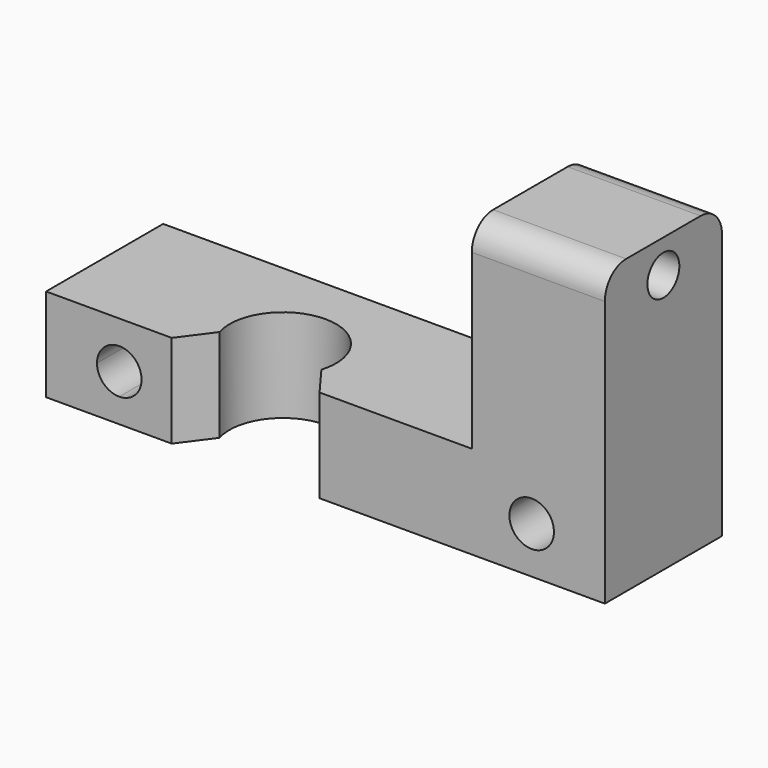
from build123d import *

# Parameters (mm, degrees)
F1_W        = 42
F1_H        = 11
F2_DEPTH    = 7
F3_R        = 4
F4_DEPTH    = 25
F5_T1_DEPTH = 25.9605224852
F7_DEPTH    = 25
F8_W        = 10
F8_H        = 11
F9_DEPTH    = 15
F10_R       = 1.5
F11_DEPTH   = 25
F12_R       = 2


# Not quite as in the source:
# - a fillet or chamfer that OpenCascade refuses, or shapes differently, is made with other operations: its cross-section is extruded or revolved along the edge and cut away or added


with BuildPart() as f2:
    # F1 (on Top) → F2 (new body)
    with BuildSketch(Plane.XY):
        with Locations((21, 5.5)):
            Rectangle(F1_W, F1_H)
    extrude(amount=F2_DEPTH)

    # F3 (on face) → F4 (cut)
    with BuildSketch(Plane.XY.offset(7)):
        with Locations((15, 3.5)):
            Circle(F3_R)
    extrude(amount=-F4_DEPTH, mode=Mode.SUBTRACT)

    # F5: chamfer of 7 on 2 edges, made by hand

    # F5_s2 → F5_t1 (cut)
    with BuildSketch(Plane.XY.offset(-9.4802612426)):
        with BuildLine():
            Line((20.721915214, -0.225000294), (18.6596772309, 2.5591704653))
            Line((18.6596772309, 2.5591704653), (18.5257555, 2.5999745093))
            ThreePointArc((18.5257555, 2.5999745093), (18.0236462707, 1.1005910665), (16.8687144645, 0.1225))
            Line((16.8687144645, 0.1225), (16.9364916731, -0.14))
            ThreePointArc((16.9364916731, -0.14), (18.8292034436, -0.14), (20.721915214, -0.365000294))
            Line((20.721915214, -0.365000294), (20.721915214, -0.225000294))
        make_face()
        with BuildLine():
            Line((11.3403227691, 2.5591704653), (9.278084786, -0.225000294))
            Line((9.278084786, -0.225000294), (9.278084786, -0.365000294))
            ThreePointArc((9.278084786, -0.365000294), (11.1707965564, -0.14), (13.0635083269, -0.14))
            Line((13.0635083269, -0.14), (13.1312855355, 0.1225))
            ThreePointArc((13.1312855355, 0.1225), (11.9763537293, 1.1005910665), (11.4742445, 2.5999745093))
            Line((11.4742445, 2.5999745093), (11.3403227691, 2.5591704653))
        make_face()
    extrude(amount=F5_T1_DEPTH, mode=Mode.SUBTRACT)

    # F6 (on face) → F7 (cut)
    with BuildSketch(Plane(origin=(0, 11, 0), x_dir=(-1, 0, 0), z_dir=(0, 1, 0))):
        with BuildLine():
            Line((-5.5, 3.5), (-3.825, 3.5))
            ThreePointArc((-3.825, 3.5), (-4.3155961415, 4.6844038585), (-5.5, 5.175))
            Line((-5.5, 5.175), (-5.5, 3.5))
        make_face()
        with BuildLine():
            ThreePointArc((-5.5, 1.825), (-4.3155961415, 2.3155961415), (-3.825, 3.5))
            Line((-3.825, 3.5), (-5.5, 3.5))
            Line((-5.5, 3.5), (-5.5, 1.825))
        make_face()
        with BuildLine():
            Line((-5.5, 3.5), (-5.5, 5.175))
            ThreePointArc((-5.5, 5.175), (-7.175, 3.5), (-5.5, 1.825))
            Line((-5.5, 1.825), (-5.5, 3.5))
        make_face()
        with BuildLine():
            ThreePointArc((-38.175, 3.5), (-36.5, 1.825), (-34.825, 3.5))
            ThreePointArc((-34.825, 3.5), (-36.5, 5.175), (-38.175, 3.5))
        make_face()
    extrude(amount=-F7_DEPTH, mode=Mode.SUBTRACT)

    # F8 (on face) → F9 (join)
    with BuildSketch(Plane.XY.offset(7)):
        with Locations((37, 5.5)):
            Rectangle(F8_W, F8_H)
    extrude(amount=F9_DEPTH)

    # F10 (on face) → F11 (cut)
    with BuildSketch(Plane.YZ.offset(42)):
        with Locations((5.5, 19.5)):
            Circle(F10_R)
    extrude(amount=-F11_DEPTH, mode=Mode.SUBTRACT)

    # F12
    f12_edges = [f2.edges().sort_by_distance(p)[0] for p in [
        (37, 0, 22),
        (37, 11, 22),
    ]]
    fillet(f12_edges, radius=F12_R)


solid = f2.part
